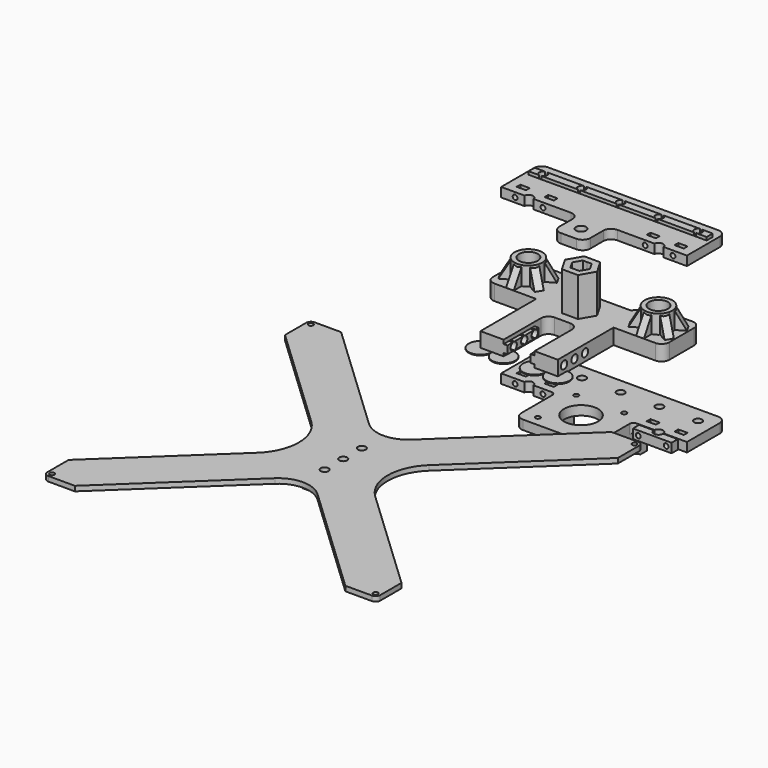
from build123d import *
from build123d import SkipClean  # not in build123d's __all__

# Parameters (mm, degrees)
F0_R             = 3.25
F1_DEPTH         = 10
F2_R             = 9
F2_R_2           = 6.05
F3_DEPTH         = 12
F5_DEPTH         = 25
F6_R             = 6.05
F7_DEPTH         = 8
F10_DEPTH        = 7
F12_DEPTH        = 2.5
F12_COPIES_COUNT = 6
F13_W            = 2.5
F13_H            = 5
F14_DEPTH        = 25
F15_R            = 2.55
F16_DEPTH        = 25
F19_R            = 3.25
F19_W            = 6
F19_H            = 3
F20_DEPTH        = 6
F21_R            = 1.55
F22_DEPTH        = 10
F23_W            = 4.9
F23_H            = 2
F24_DEPTH        = 57.5
F25_R            = 2.55
F26_DEPTH        = 10
F28_R            = 1.55
F28_R_2          = 11
F28_W            = 6
F28_H            = 3
F29_DEPTH        = 6
F30_R            = 1.55
F31_DEPTH        = 10
F32_W            = 4.9
F32_H            = 2
F33_DEPTH        = 57.5
F34_R            = 2.55
F35_DEPTH        = 10
F37_DEPTH        = 3
F40_DEPTH        = 6
F41_R            = 1.55
F42_DEPTH        = 6
F43_R            = 1.55
F43_R_2          = 2.55
F44_DEPTH        = 3.175
F45_W            = 5
F45_H            = 5
F46_DEPTH        = 2
F48_DEPTH        = 0.5


# Not quite as in the source:
# - a pattern or mirror of a feature is missing from the dataset's text; its kind, count and spacing are read off the source's solid


with BuildPart() as f1:
    # F0 (on Top) → F1 (new body)
    with BuildSketch(Plane.XY):
        with BuildLine():
            ThreePointArc((0, 3.25), (3.25, 0), (0, -3.25))
            Line((0, -3.25), (0, -15))
            Line((0, -15), (5, -15))
            ThreePointArc((5, -15), (8.5355339059, -16.4644660941), (10, -20))
            Line((10, -20), (10, -50))
            Line((10, -50), (25, -50))
            Line((25, -50), (25, -5))
            Line((25, -5), (52, -5))
            ThreePointArc((52, -5), (55.5355339059, -3.5355339059), (57, 0))
            Line((57, 0), (57, 20))
            ThreePointArc((57, 20), (55.5355339059, 23.5355339059), (52, 25))
            Line((52, 25), (30, 25))
            Line((30, 25), (20, 15))
            Line((20, 15), (0, 15))
            Line((0, 15), (0, 3.25))
        make_face()
        with Locations((42, 10)):
            Circle(F0_R, mode=Mode.SUBTRACT)
    extrude(amount=F1_DEPTH)

    # F2 (on face) → F3 (join)
    with BuildSketch(Plane.XY.offset(10)):
        with Locations((42, 10)):
            Circle(F2_R)
        with Locations((42, 10)):
            Circle(F2_R_2, mode=Mode.SUBTRACT)
    extrude(amount=F3_DEPTH)

    # F4 (on face) → F5 (join)
    with BuildSketch(Plane.XY.offset(10)):
        Polygon((0, 9), (0, 5), (2.8867513459, 5), (5.7735026919, 0), (2.8867513459, -5), (0, -5), (0, -9), (5.1961524227, -9), (10.3923048454, 0), (5.1961524227, 9), align=None)
    extrude(amount=F5_DEPTH)

    # F6 (on face) → F7 (cut)
    with BuildSketch(Plane.XY.offset(10)):
        with Locations((42, 10)):
            Circle(F6_R)
    extrude(amount=-F7_DEPTH, mode=Mode.SUBTRACT)

    # F9 (on face) → F10 (cut)
    with BuildSketch(Plane(origin=(0, 0, 0), x_dir=(1, 0, 0), z_dir=(0, 0, -1))):
        with BuildLine():
            Line((2.8867513459, 5), (0, 5))
            Line((0, 5), (0, 3.25))
            ThreePointArc((0, 3.25), (3.25, 0), (0, -3.25))
            Line((0, -3.25), (0, -5))
            Line((0, -5), (2.8867513459, -5))
            Line((2.8867513459, -5), (5.7735026919, 0))
            Line((5.7735026919, 0), (2.8867513459, 5))
        make_face()
    extrude(amount=-F10_DEPTH, mode=Mode.SUBTRACT)

    # F11 (on offset) → F12 (join, symmetric)
    with BuildSketch(Plane.YZ.offset(42)):
        Polygon((2, 10), (2, 22), (-4.9282032303, 10), align=None)
    f12 = extrude(amount=F12_DEPTH, both=True)

    # F12_copies: F12 ×6 about axis
    f12_copies_axis = Axis((42, 10, 0), (0, 0, 1))
    for i in range(1, F12_COPIES_COUNT):
        add(f12.rotate(f12_copies_axis, i * 360 / F12_COPIES_COUNT), clean=False)

    # F13 (on face) → F14 (join)
    with BuildSketch(Plane.XZ.offset(50)):
        with Locations((8.75, 5)):
            Rectangle(F13_W, F13_H)
    extrude(amount=-F14_DEPTH)

    # F15 (on face) → F16 (cut)
    with BuildSketch(Plane(origin=(7.5, 0, 0), x_dir=(0, -1, 0), z_dir=(-1, 0, 0))):
        with Locations((45, 5)):
            Circle(F15_R)
        with Locations((36.5, 5)):
            Circle(F15_R)
        with Locations((28, 5)):
            Circle(F15_R)
    extrude(amount=-F16_DEPTH, mode=Mode.SUBTRACT)

    # F17: F1 across plane


with BuildPart() as f1_1:
    add(f1.part, clean=False)
    with SkipClean():  # cleaning this boolean's faces spoils the solid; the shape is the same uncleaned
        add(f1.part.mirror(Plane.YZ), clean=False)

    # F47 (on face) → F48 (join)
    with BuildSketch(Plane(origin=(0, 0, 0), x_dir=(1, 0, 0), z_dir=(0, 0, -1))):
        with BuildLine():
            Line((25, 50), (25, 42.5))
            ThreePointArc((25, 42.5), (30.3033008589, 55.3033008589), (17.5, 50))
            Line((17.5, 50), (25, 50))
        make_face()
        with BuildLine():
            Line((10, 50), (17.5, 50))
            ThreePointArc((17.5, 50), (4.6966991411, 55.3033008589), (10, 42.5))
            Line((10, 42.5), (10, 50))
        make_face()
        with BuildLine():
            Line((-10, 50), (-10, 42.5))
            ThreePointArc((-10, 42.5), (-4.6966991411, 55.3033008589), (-17.5, 50))
            Line((-17.5, 50), (-10, 50))
        make_face()
        with BuildLine():
            Line((-25, 50), (-17.5, 50))
            ThreePointArc((-17.5, 50), (-30.3033008589, 55.3033008589), (-25, 42.5))
            Line((-25, 42.5), (-25, 50))
        make_face()
    extrude(amount=-F48_DEPTH)


with BuildPart() as f20:
    # F19 (on offset) → F20 (new body)
    with BuildSketch(Plane.XY.offset(50)):
        with BuildLine():
            ThreePointArc((-44.9580398915, 10.5), (-42, 13), (-39.0419601085, 10.5))
            Line((-39.0419601085, 10.5), (-15, 10.5))
            ThreePointArc((-15, 10.5), (-11.4644660941, 9.0355339059), (-10, 5.5))
            Line((-10, 5.5), (-10, -5))
            ThreePointArc((-10, -5), (-8.5355339059, -8.5355339059), (-5, -10))
            Line((-5, -10), (5, -10))
            ThreePointArc((5, -10), (8.5355339059, -8.5355339059), (10, -5))
            Line((10, -5), (10, 5.5))
            ThreePointArc((10, 5.5), (11.4644660941, 9.0355339059), (15, 10.5))
            Line((15, 10.5), (39.0419601085, 10.5))
            ThreePointArc((39.0419601085, 10.5), (42, 13), (44.9580398915, 10.5))
            Line((44.9580398915, 10.5), (60, 10.5))
            Line((60, 10.5), (60, 37))
            ThreePointArc((60, 37), (58.5355339059, 40.5355339059), (55, 42))
            Line((55, 42), (-55, 42))
            ThreePointArc((-55, 42), (-58.5355339059, 40.5355339059), (-60, 37))
            Line((-60, 37), (-60, 10.5))
            Line((-60, 10.5), (-44.9580398915, 10.5))
        make_face()
        Circle(F19_R, mode=Mode.SUBTRACT)
        with Locations((-51, 17)):
            Rectangle(F19_W, F19_H, mode=Mode.SUBTRACT)
        with Locations((-33, 17)):
            Rectangle(F19_W, F19_H, mode=Mode.SUBTRACT)
        with Locations((33, 17)):
            Rectangle(F19_W, F19_H, mode=Mode.SUBTRACT)
        with Locations((51, 17)):
            Rectangle(F19_W, F19_H, mode=Mode.SUBTRACT)
    extrude(amount=F20_DEPTH)

    # F21 (on face) → F22 (cut)
    with BuildSketch(Plane(origin=(0, 15.5, 0), x_dir=(-1, 0, 0), z_dir=(0, 1, 0))):
        with Locations((51, 53)):
            Circle(F21_R)
        with Locations((33, 53)):
            Circle(F21_R)
        with Locations((-33, 53)):
            Circle(F21_R)
        with Locations((-51, 53)):
            Circle(F21_R)
    extrude(amount=-F22_DEPTH, mode=Mode.SUBTRACT)

    # F23 (on Right) → F24 (join, symmetric)
    with BuildSketch(Plane.YZ):
        with Locations((32, 57)):
            Rectangle(F23_W, F23_H)
    extrude(amount=F24_DEPTH, both=True)

    # F25 (on face) → F26 (cut)
    with BuildSketch(Plane.XY.offset(58)):
        with Locations((0, 32)):
            Circle(F25_R)
        with Locations((25, 32)):
            Circle(F25_R)
        with Locations((50, 32)):
            Circle(F25_R)
        with Locations((-25, 32)):
            Circle(F25_R)
        with Locations((-50, 32)):
            Circle(F25_R)
    extrude(amount=-F26_DEPTH, mode=Mode.SUBTRACT)


with BuildPart() as f29:
    # F28 (on offset) → F29 (new body)
    with BuildSketch(Plane.XY.offset(-50)):
        with BuildLine():
            ThreePointArc((-44.9580398915, 10.5), (-42, 13), (-39.0419601085, 10.5))
            Line((-39.0419601085, 10.5), (-27.5, 10.5))
            ThreePointArc((-27.5, 10.5), (-25.732233047, 9.767766953), (-25, 8))
            Line((-25, 8), (-25, -17))
            ThreePointArc((-25, -17), (-23.5355339059, -20.5355339059), (-20, -22))
            Line((-20, -22), (20, -22))
            ThreePointArc((20, -22), (23.5355339059, -20.5355339059), (25, -17))
            Line((25, -17), (25, 8))
            ThreePointArc((25, 8), (25.732233047, 9.767766953), (27.5, 10.5))
            Line((27.5, 10.5), (39.0419601085, 10.5))
            ThreePointArc((39.0419601085, 10.5), (42, 13), (44.9580398915, 10.5))
            Line((44.9580398915, 10.5), (60, 10.5))
            Line((60, 10.5), (60, 37))
            ThreePointArc((60, 37), (58.5355339059, 40.5355339059), (55, 42))
            Line((55, 42), (-55, 42))
            ThreePointArc((-55, 42), (-58.5355339059, 40.5355339059), (-60, 37))
            Line((-60, 37), (-60, 10.5))
            Line((-60, 10.5), (-44.9580398915, 10.5))
        make_face()
        with Locations((-15.5, -15.5)):
            Circle(F28_R, mode=Mode.SUBTRACT)
        with Locations((15.5, -15.5)):
            Circle(F28_R, mode=Mode.SUBTRACT)
        Circle(F28_R_2, mode=Mode.SUBTRACT)
        with Locations((-51, 17)):
            Rectangle(F28_W, F28_H, mode=Mode.SUBTRACT)
        with Locations((-33, 17)):
            Rectangle(F28_W, F28_H, mode=Mode.SUBTRACT)
        with Locations((-15.5, 15.5)):
            Circle(F28_R, mode=Mode.SUBTRACT)
        with Locations((15.5, 15.5)):
            Circle(F28_R, mode=Mode.SUBTRACT)
        with Locations((33, 17)):
            Rectangle(F28_W, F28_H, mode=Mode.SUBTRACT)
        with Locations((51, 17)):
            Rectangle(F28_W, F28_H, mode=Mode.SUBTRACT)
    extrude(amount=-F29_DEPTH)

    # F30 (on face) → F31 (cut)
    with BuildSketch(Plane(origin=(0, 15.5, 0), x_dir=(-1, 0, 0), z_dir=(0, 1, 0))):
        with Locations((51, -53)):
            Circle(F30_R)
        with Locations((33, -53)):
            Circle(F30_R)
        with Locations((-33, -53)):
            Circle(F30_R)
        with Locations((-51, -53)):
            Circle(F30_R)
    extrude(amount=-F31_DEPTH, mode=Mode.SUBTRACT)

    # F32 (on Right) → F33 (join, symmetric)
    with BuildSketch(Plane.YZ):
        with Locations((32, -57)):
            Rectangle(F32_W, F32_H)
    extrude(amount=F33_DEPTH, both=True)

    # F34 (on face) → F35 (cut)
    with BuildSketch(Plane.XY.offset(-50)):
        with Locations((-50, 32)):
            Circle(F34_R)
        with Locations((-25, 32)):
            Circle(F34_R)
        with Locations((0, 32)):
            Circle(F34_R)
        with Locations((25, 32)):
            Circle(F34_R)
        with Locations((50, 32)):
            Circle(F34_R)
    extrude(amount=-F35_DEPTH, mode=Mode.SUBTRACT)

    # F36 (on face) → F37 (join)
    with BuildSketch(Plane.YZ.offset(25)):
        Polygon((21.9, -56), (-16.1, -56), (16.9, -71), (21.9, -71), align=None)
    extrude(amount=-F37_DEPTH)

    # F38: F29 across plane


with BuildPart() as f29_1:
    add(f29.part, clean=False)
    add(f29.part.mirror(Plane.YZ), clean=False)


with BuildPart() as f40:
    # F39 (on face) → F40 (new body)
    with BuildSketch(Plane.XY.offset(-50)):
        with BuildLine():
            ThreePointArc((45, 10), (42, 7), (39, 10))
            Line((39, 10), (29.5, 10))
            Line((29.5, 10), (29.5, 5))
            Line((29.5, 5), (54.5, 5))
            Line((54.5, 5), (54.5, 10))
            Line((54.5, 10), (45, 10))
        make_face()
    extrude(amount=-F40_DEPTH)

    # F41 (on face) → F42 (cut)
    with BuildSketch(Plane.XZ.offset(-5)):
        with Locations((33, -53)):
            Circle(F41_R)
        with Locations((51, -53)):
            Circle(F41_R)
    extrude(amount=-F42_DEPTH, mode=Mode.SUBTRACT)


with BuildPart() as f44:
    # F43 (on Top) → F44 (new body)
    with BuildSketch(Plane.XY):
        with BuildLine():
            Line((104.5, -84.5027588444), (87.3570260483, -84.5027588444))
            Line((87.3570260483, -84.5027588444), (13.7321312465, -154.0341302282))
            ThreePointArc((13.7321312465, -154.0341302282), (0, -159.4935466282), (-13.7321312465, -154.0341302282))
            Line((-13.7321312465, -154.0341302282), (-87.3570260483, -84.5027588444))
            Line((-87.3570260483, -84.5027588444), (-104.5, -84.5027588444))
            ThreePointArc((-104.5, -84.5027588444), (-106.6213203436, -85.3814385008), (-107.5, -87.5027588444))
            Line((-107.5, -87.5027588444), (-107.5, -104.6457327961))
            Line((-107.5, -104.6457327961), (-38.0949480055, -170.1918834444))
            ThreePointArc((-38.0949480055, -170.1918834444), (-28.6931448753, -192.0027588444), (-38.0949480055, -213.8136342444))
            Line((-38.0949480055, -213.8136342444), (-107.5, -279.3597848927))
            Line((-107.5, -279.3597848927), (-107.5, -296.5027588444))
            ThreePointArc((-107.5, -296.5027588444), (-106.6213203436, -298.6240791879), (-104.5, -299.5027588444))
            Line((-104.5, -299.5027588444), (-87.3570260483, -299.5027588444))
            Line((-87.3570260483, -299.5027588444), (-13.7321312465, -229.9713874606))
            ThreePointArc((-13.7321312465, -229.9713874606), (0, -224.5119710606), (13.7321312465, -229.9713874606))
            Line((13.7321312465, -229.9713874606), (87.3570260483, -299.5027588444))
            Line((87.3570260483, -299.5027588444), (104.5, -299.5027588444))
            ThreePointArc((104.5, -299.5027588444), (106.6213203436, -298.6240791879), (107.5, -296.5027588444))
            Line((107.5, -296.5027588444), (107.5, -279.3597848927))
            Line((107.5, -279.3597848927), (38.0949480055, -213.8136342444))
            ThreePointArc((38.0949480055, -213.8136342444), (28.6931448753, -192.0027588444), (38.0949480055, -170.1918834444))
            Line((38.0949480055, -170.1918834444), (107.5, -104.6457327961))
            Line((107.5, -104.6457327961), (107.5, -87.5027588444))
            ThreePointArc((107.5, -87.5027588444), (106.6213203436, -85.3814385008), (104.5, -84.5027588444))
        make_face()
        with Locations((-104.5, -296.5027588444)):
            Circle(F43_R, mode=Mode.SUBTRACT)
        with Locations((104.5, -296.5027588444)):
            Circle(F43_R, mode=Mode.SUBTRACT)
        with Locations((0, -207.0027588444)):
            Circle(F43_R_2, mode=Mode.SUBTRACT)
        with Locations((-104.5, -87.5027588444)):
            Circle(F43_R, mode=Mode.SUBTRACT)
        with Locations((0, -192.0027588444)):
            Circle(F43_R_2, mode=Mode.SUBTRACT)
        with Locations((0, -177.0027588444)):
            Circle(F43_R_2, mode=Mode.SUBTRACT)
        with Locations((104.5, -87.5027588444)):
            Circle(F43_R, mode=Mode.SUBTRACT)
    extrude(amount=F44_DEPTH)

    # F45 (on face) → F46 (join)
    with BuildSketch(Plane(origin=(0, 0, 0), x_dir=(1, 0, 0), z_dir=(0, 0, -1))):
        with Locations((0, 219.5527588444)):
            Rectangle(F45_W, F45_H)
    extrude(amount=F46_DEPTH)


solid = Compound([f1_1.part, f20.part, f29_1.part, f40.part, f44.part])
